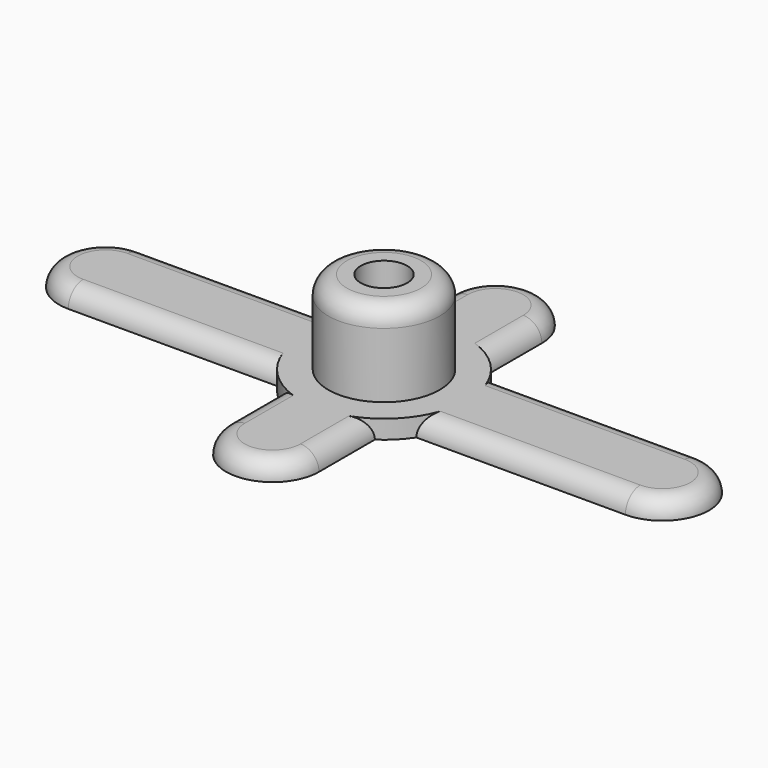
from build123d import *

# Parameters (mm, degrees)
F0_R     = 2.5
F1_DEPTH = 2
F2_R     = 6
F2_R_2   = 2.5
F3_DEPTH = 9
F4_R     = 2
F5_R     = 1.99999


# Not quite as in the source:
# - a fillet or chamfer is up to 0.001 mm smaller than in the source, because OpenCascade refuses the exact size


with BuildPart() as f1:
    # F0 (on Top) → F1 (new body)
    with BuildSketch(Plane.XY):
        with BuildLine():
            Line((-30, -5), (-7.4833147735, -5))
            ThreePointArc((-7.4833147735, -5), (-6.3639610307, -6.3639610307), (-5, -7.4833147735))
            Line((-5, -7.4833147735), (-5, -15))
            ThreePointArc((-5, -15), (0, -20), (5, -15))
            Line((5, -15), (5, -7.4833147735))
            ThreePointArc((5, -7.4833147735), (6.3639610307, -6.3639610307), (7.4833147735, -5))
            Line((7.4833147735, -5), (30, -5))
            ThreePointArc((30, -5), (35, 0), (30, 5))
            Line((30, 5), (7.4833147735, 5))
            ThreePointArc((7.4833147735, 5), (6.3639610307, 6.3639610307), (5, 7.4833147735))
            Line((5, 7.4833147735), (5, 15))
            ThreePointArc((5, 15), (0, 20), (-5, 15))
            Line((-5, 15), (-5, 7.4833147735))
            ThreePointArc((-5, 7.4833147735), (-6.3639610307, 6.3639610307), (-7.4833147735, 5))
            Line((-7.4833147735, 5), (-30, 5))
            ThreePointArc((-30, 5), (-35, 0), (-30, -5))
        make_face()
        Circle(F0_R, mode=Mode.SUBTRACT)
    extrude(amount=F1_DEPTH)

    # F2 (on face) → F3 (join)
    with BuildSketch(Plane.XY.offset(2)):
        Circle(F2_R)
        Circle(F2_R_2, mode=Mode.SUBTRACT)
    extrude(amount=F3_DEPTH)

    # F4
    f4_edges = [f1.edges().sort_by_distance(p)[0] for p in [
        (-6, 0, 11),
    ]]
    fillet(f4_edges, radius=F4_R)

    # F5 (radius 2 in the source; OpenCascade refuses exactly that, so slightly less here)
    f5_edges = [f1.edges().sort_by_distance(p)[0] for p in [
        (35, 0, 2),
        (0, 20, 2),
        (0, -20, 2),
        (-35, 0, 2),
    ]]
    fillet(f5_edges, radius=F5_R)


solid = f1.part
